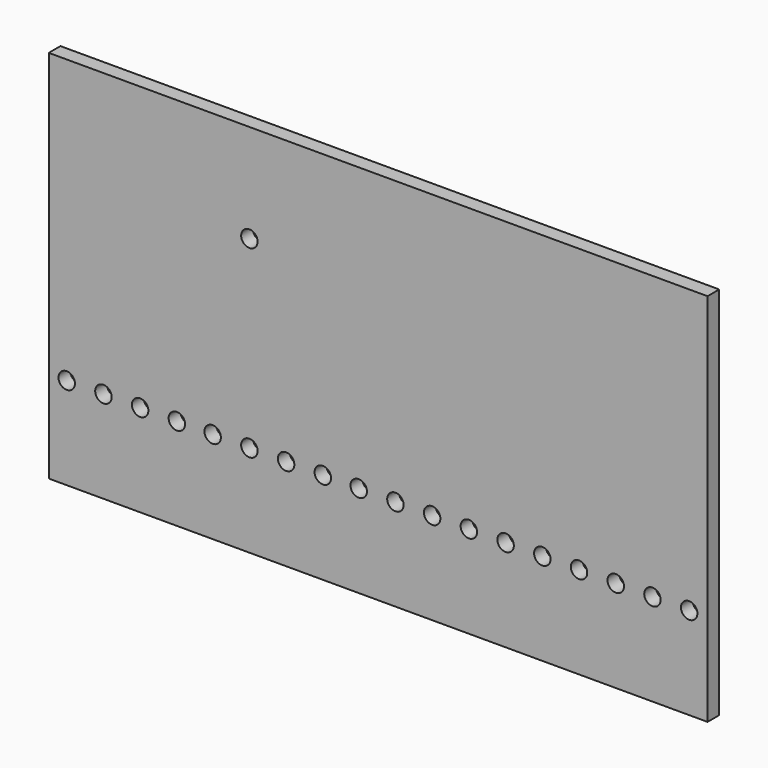
from build123d import *

# Parameters (mm, degrees)
F0_R     = 1.7859375
F1_DEPTH = 3.175


# Not quite as in the source:
# - a length typed as a fraction of an inch, garbled in the dataset ("3 / 203.2 mm" for 3/8 in), is restored


with BuildPart() as f1:
    # F0 (on Front) → F1 (new body)
    with BuildSketch(Plane.XZ):
        Polygon((75.715, -20), (75.715, 61.3500024), (-3.7115799668, 61.3500024), (-35.4027799668, 61.3500024), (-67.2774, 61.3500024), (-67.2774, -20), (-35.5862, -20), (-3.895, -20), align=None)
        with Locations((-63.3824, 0)):
            Circle(F0_R, mode=Mode.SUBTRACT)
        with Locations((-55.4124, 0)):
            Circle(F0_R, mode=Mode.SUBTRACT)
        with Locations((-47.4424, 0)):
            Circle(F0_R, mode=Mode.SUBTRACT)
        with Locations((-39.4724, 0)):
            Circle(F0_R, mode=Mode.SUBTRACT)
        with Locations((-31.7, 0)):
            Circle(F0_R, mode=Mode.SUBTRACT)
        with Locations((-23.73, 0)):
            Circle(F0_R, mode=Mode.SUBTRACT)
        with Locations((-15.76, 0)):
            Circle(F0_R, mode=Mode.SUBTRACT)
        with Locations((-7.79, 0)):
            Circle(F0_R, mode=Mode.SUBTRACT)
        Circle(F0_R, mode=Mode.SUBTRACT)
        with Locations((7.97, 0)):
            Circle(F0_R, mode=Mode.SUBTRACT)
        with Locations((15.94, 0)):
            Circle(F0_R, mode=Mode.SUBTRACT)
        with Locations((23.91, 0)):
            Circle(F0_R, mode=Mode.SUBTRACT)
        with Locations((31.88, 0)):
            Circle(F0_R, mode=Mode.SUBTRACT)
        with Locations((39.85, 0)):
            Circle(F0_R, mode=Mode.SUBTRACT)
        with Locations((47.82, 0)):
            Circle(F0_R, mode=Mode.SUBTRACT)
        with Locations((55.79, 0)):
            Circle(F0_R, mode=Mode.SUBTRACT)
        with Locations((63.76, 0)):
            Circle(F0_R, mode=Mode.SUBTRACT)
        with Locations((71.73, 0)):
            Circle(F0_R, mode=Mode.SUBTRACT)
        with Locations((-23.73, 40.005)):
            Circle(F0_R, mode=Mode.SUBTRACT)
    extrude(amount=F1_DEPTH)


solid = f1.part
